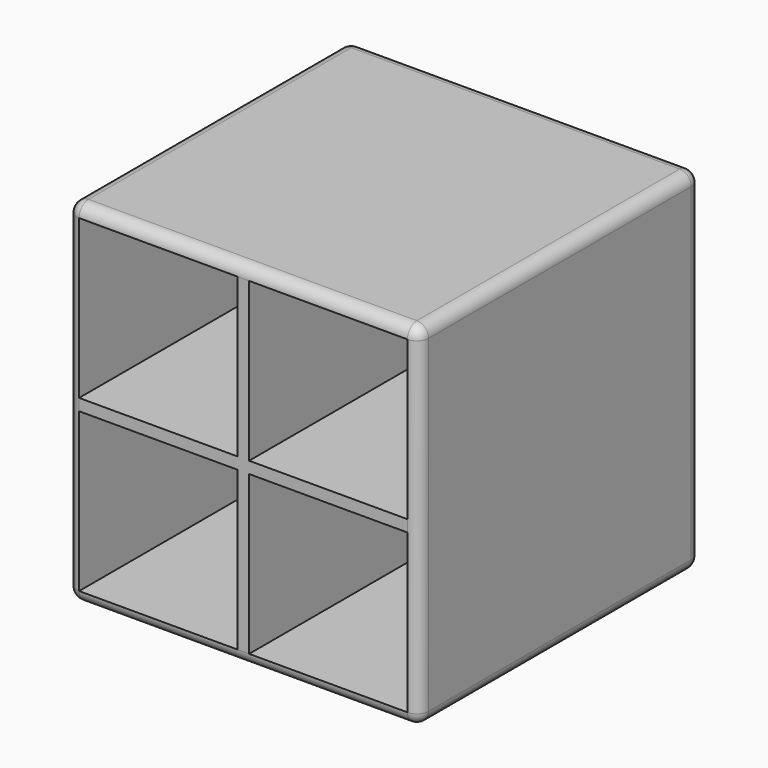
from build123d import *

# Parameters (mm, degrees)
F0_W     = 150
F0_H     = 150
F0_W_2   = 67.5
F0_H_2   = 67.5
F1_DEPTH = 150
F2_R     = 5
F3_R     = 4.99999


# Not quite as in the source:
# - a fillet or chamfer is up to 0.001 mm smaller than in the source, because OpenCascade refuses the exact size


with BuildPart() as f1:
    # F0 (on Front) → F1 (new body)
    with BuildSketch(Plane.XZ):
        with Locations((75, 75)):
            Rectangle(F0_W, F0_H)
        with Locations((38.75, 38.75)):
            Rectangle(F0_W_2, F0_H_2, mode=Mode.SUBTRACT)
        with Locations((111.25, 38.75)):
            Rectangle(F0_W_2, F0_H_2, mode=Mode.SUBTRACT)
        with Locations((38.75, 111.25)):
            Rectangle(F0_W_2, F0_H_2, mode=Mode.SUBTRACT)
        with Locations((111.25, 111.25)):
            Rectangle(F0_W_2, F0_H_2, mode=Mode.SUBTRACT)
    extrude(amount=F1_DEPTH)

    # F2
    f2_edges = [f1.edges().sort_by_distance(p)[0] for p in [
        (150, -75, 150),
    ]]
    fillet(f2_edges, radius=F2_R)

    # F3 (radius 5 in the source; OpenCascade refuses exactly that, so slightly less here)
    f3_edges = [f1.edges().sort_by_distance(p)[0] for p in [
        (72.5, -150, 150),
        (150, -150, 72.5),
        (72.5, 0, 150),
        (0, -75, 150),
        (75, -150, 0),
        (150, -75, 0),
        (0, -150, 75),
        (150, 0, 72.5),
        (0, 0, 75),
        (0, -75, 0),
        (75, 0, 0),
    ]]
    fillet(f3_edges, radius=F3_R)


solid = f1.part
